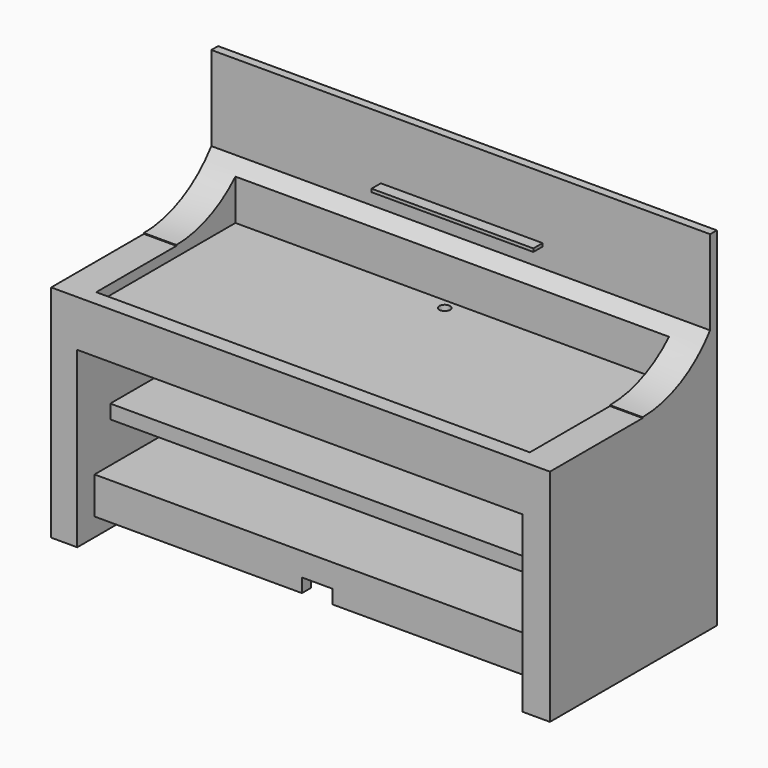
from build123d import *

# Parameters (mm, degrees)
F0_W          = 109.3183457851
F0_H          = 33.4434658289
F1_DEPTH      = 45.72
F2_W          = 95.0407683849
F2_H          = 38.138333708
F3_DEPTH      = 25.4
F4_W          = 109.3183457851
F4_H          = 23.2531316578
F5_DEPTH      = 25.4
F7_DEPTH      = 254
F9_W          = 5.9644132853
F9_H          = 45.72
F9_W_2        = 5.7119317353
F10_DEPTH     = 38.1
F11_W         = 29.130092822
F11_H         = 3.0559636652
F12_DEPTH     = 101.6
F14_DEPTH     = 127
F15_DEPTH     = 18.5456499457
F16_W         = 35.4631710798
F16_H         = 0.6852131337
F17_DEPTH     = 2.54
F18_W         = 38.6509299278
F18_H         = 8.1171598285
F19_DEPTH     = 99.9768525362
F20_T         = 2.54
F20_T3_DEPTH  = 114.3983457851
F20_T5_DEPTH  = 40.5431710798
F20_T7_DEPTH  = 5.7652131337
F20_T9_DEPTH  = 12.2003224361
F20_T11_DEPTH = 12.2372549641
F20_T13_DEPTH = 50.8
F20_T15_DEPTH = 13.1971598285
F20_T17_DEPTH = 43.7309299278
F20_T19_DEPTH = 34.210092822
F20_T21_DEPTH = 8.1359636652
F20_T23_DEPTH = 7.2268683422
F20_T25_DEPTH = 43.218333708
F20_T27_DEPTH = 14.0249238314
F20_T29_DEPTH = 100.1207683849
F21_W         = 6.7161731422
F21_H         = 3.0271708965
F22_DEPTH     = 25.4
F8_R          = 1.1732121366
F23_DEPTH     = 69.3976804614


# Not quite as in the source:
# - a shell that OpenCascade refuses in one call is made with other operations: the cavity is built on its own and cut out


with BuildPart() as f1:
    # F0 (on Front) → F1 (new body)
    with BuildSketch(Plane.XZ):
        with Locations((-0.1045018435, 16.7217329144)):
            Rectangle(F0_W, F0_H)
    extrude(amount=F1_DEPTH)

    # F2 (on face) → F3 (cut)
    with BuildSketch(Plane.XY.offset(33.4434658289)):
        with Locations((-0.1229681075, -23.2116412371)):
            Rectangle(F2_W, F2_H)
    extrude(amount=-F3_DEPTH, mode=Mode.SUBTRACT)

    # F4 (on face) → F5 (cut)
    with BuildSketch(Plane.XZ.offset(45.72)):
        with Locations((-0.1045018435, 21.8169)):
            Rectangle(F4_W, F4_H)
    extrude(amount=-F5_DEPTH, mode=Mode.SUBTRACT)

    # F6 (on face) → F7 (cut)
    with BuildSketch(Plane.YZ.offset(54.5546710491)):
        with BuildLine():
            Line((-20.32, 33.4434658289), (-20.32, 10.3678972162))
            ThreePointArc((-20.32, 10.3678972162), (-8.4847772871, 13.6341404962), (0, 22.5082261516))
            Line((0, 22.5082261516), (0, 33.4434658289))
            Line((0, 33.4434658289), (-20.32, 33.4434658289))
        make_face()
        with BuildLine():
            ThreePointArc((0, 22.5082261516), (2.0560745106, 27.8049237926), (2.7555686127, 33.4434658289))
            ThreePointArc((2.7555686127, 33.4434658289), (-36.6368910458, 49.7603568747), (-20.32, 10.3678972162))
            Line((-20.32, 10.3678972162), (-20.32, 33.4434658289))
            Line((-20.32, 33.4434658289), (0, 33.4434658289))
            Line((0, 33.4434658289), (0, 22.5082261516))
        make_face()
    extrude(amount=-F7_DEPTH, mode=Mode.SUBTRACT)

    # F9 (on face) → F10 (join)
    with BuildSketch(Plane(origin=(0, 0, 0), x_dir=(1, 0, 0), z_dir=(0, 0, -1))):
        with Locations((51.5724644065, 22.86)):
            Rectangle(F9_W, F9_H)
        with Locations((-51.9077088684, 22.86)):
            Rectangle(F9_W_2, F9_H)
    extrude(amount=F10_DEPTH)

    # F11 (on face) → F12 (join)
    with BuildSketch(Plane.YZ.offset(-49.0517430007)):
        with Locations((-22.1103844233, -15.5687723309)):
            Rectangle(F11_W, F11_H)
    extrude(amount=F12_DEPTH)

    # F13 (on face) → F14 (cut)
    with BuildSketch(Plane.YZ.offset(54.5546710491)):
        with BuildLine():
            ThreePointArc((0, 22.5082261516), (-0.8668457158, 21.0315096899), (-1.8408102843, 19.6231397021))
            Line((-1.8408102843, 19.6231397021), (0, 19.6231397021))
            Line((0, 19.6231397021), (0, 22.5082261516))
        make_face()
    extrude(amount=-F14_DEPTH, mode=Mode.SUBTRACT)

    # F15 (add): a face of the model
    f15_faces = [f1.faces().sort_by_distance(p)[0] for p in [
        (-0.1045018435, -0.9204051421, 19.6231397021),
    ]]
    extrude(f15_faces, amount=F15_DEPTH)

    # F16 (on face) → F17 (join)
    with BuildSketch(Plane.XZ.offset(1.8408102843)):
        with Locations((0.1093326136, 24.1770995781)):
            Rectangle(F16_W, F16_H)
    extrude(amount=F17_DEPTH)

    # F18 (on face) → F19 (join)
    with BuildSketch(Plane(origin=(48.5902577639, 0, 0), x_dir=(0, -1, 0), z_dir=(-1, 0, 0))):
        with Locations((21.6686017811, -30.0215007737)):
            Rectangle(F18_W, F18_H)
    extrude(amount=F19_DEPTH)

    # F20: shell of thickness 2.54, made by hand


with BuildPart() as f20_core1:
    # F20_t2: copy of F1
    add(f1.part)

    # the walls: a layer under each face that stays
    f20_faces = [f20_core1.faces().sort_by_distance(p)[0] for p in [
        (-54.763674736, -22.86, 0.0343948239),
        (-0.1045018435, 0, 0.0343948239),
        (-0.1045018435, -0.9204051421, 38.1687896479),
        (-0.1045018435, -1.8408102843, 28.895964675),
        (-46.9552214657, -2.7975084588, 18.4286678952),
        (-51.203513518, -20.32, 10.2791156936),
        (-46.9552214657, -43.9057142857, 10.1903341711),
        (-36.5439504385, -45.72, 2.1419451425),
        (-51.9077088684, -22.86, -38.1),
        (54.5546710491, -22.86, 0.0343948239),
        (-49.0517430007, -22.86, -19.05),
        (-0.2307426184, -22.86, 0),
        (48.5902577639, -22.86, -19.05),
        (51.5724644065, -22.86, -38.1),
        (0.1093326136, -3.1108102843, 24.5197061449),
        (-17.6222529262, -3.1108102843, 24.1770995781),
        (0.1093326136, -3.1108102843, 23.8344930112),
        (17.8409181535, -3.1108102843, 24.1770995781),
        (-47.6433522999, -10.4988633345, 9.5342864675),
        (-0.1229681075, -4.1424743831, 12.5159277446),
        (47.397416085, -35.9244191398, 9.5342864675),
        (50.9760435671, -20.32, 10.2791156936),
        (-0.1229681075, -42.2808080912, 9.1169),
        (-0.2307426184, -40.994066745, -30.0215007737),
        (-0.2307426184, -21.6686017811, -25.9629208595),
        (-0.2307426184, -2.3431368172, -30.0215007737),
        (-0.2307426184, -22.1103844233, -14.0407904983),
        (-0.2307426184, -7.5453380123, -15.5687723309),
        (-0.2307426184, -36.6754308343, -15.5687723309),
        (-0.2307426184, -22.1103844233, -17.0967541635),
        (0.1093326136, -4.3808102843, 24.1770995781),
        (-0.1229681075, -23.2116412371, 8.0434658289),
    ]]
    thicken(f20_faces, amount=-F20_T, mode=Mode.SUBTRACT)

    # F20_s4 → F20_t3 (cut)
    with BuildSketch(Plane.YZ.offset(-57.303674736)):
        Polygon((-1.8865509063, 19.6383521673), (0.6991897157, 19.6231397021), (0.6991897157, 18.7783837759), (0.1932519166, 18.1018931859), align=None)
    extrude(amount=F20_T3_DEPTH, mode=Mode.SUBTRACT)

    # F20_s6 → F20_t5 (cut)
    with BuildSketch(Plane.YZ.offset(-20.1622529262)):
        Polygon((-1.8662102843, 24.5451061449), (0.6991897157, 24.5197061449), (0.6991897157, 21.9797061449), (-1.8408102843, 21.9797061449), align=None)
        Polygon((-1.8662102843, 23.8090930112), (0.6991897157, 23.8344930112), (0.6991897157, 26.3744930112), (-1.8408102843, 26.3744930112), align=None)
    extrude(amount=F20_T5_DEPTH, mode=Mode.SUBTRACT)

    # F20_s8 → F20_t7 (cut)
    with BuildSketch(Plane.XY.offset(21.2944930112)):
        Polygon((-17.6476529262, -1.8662102843), (-17.6222529262, 0.6991897157), (-15.0822529262, 0.6991897157), (-15.0822529262, -1.8408102843), align=None)
        Polygon((17.8663181535, -1.8662102843), (17.8409181535, 0.6991897157), (15.3009181535, 0.6991897157), (15.3009181535, -1.8408102843), align=None)
    extrude(amount=F20_T7_DEPTH, mode=Mode.SUBTRACT)

    # F20_s10 → F20_t9 (cut)
    with BuildSketch(Plane.YZ.offset(-57.303674736)):
        Polygon((-20.3454, 10.2157341711), (-17.78, 10.1903341711), (-17.78, 7.6503341711), (-20.32, 7.6503341711), align=None)
    extrude(amount=F20_T9_DEPTH, mode=Mode.SUBTRACT)

    # F20_s12 → F20_t11 (cut)
    with BuildSketch(Plane.YZ.offset(44.857416085)):
        Polygon((-20.3454, 10.2157341711), (-20.32, 7.6503341711), (-17.78, 7.6503341711), (-17.78, 10.1903341711), align=None)
    extrude(amount=F20_T11_DEPTH, mode=Mode.SUBTRACT)

    # F20_s14 → F20_t13 (cut)
    with BuildSketch(Plane.XZ.offset(-2.54)):
        Polygon((-49.0263430007, -0.0254), (-51.5917430007, 0), (-51.5917430007, 2.54), (-49.0517430007, 2.54), align=None)
        Polygon((48.5648577639, -0.0254), (48.5902577639, 2.54), (51.1302577639, 2.54), (51.1302577639, 0), align=None)
    extrude(amount=F20_T13_DEPTH, mode=Mode.SUBTRACT)

    # F20_s16 → F20_t15 (cut)
    with BuildSketch(Plane.XY.offset(-36.620080688)):
        Polygon((-49.0263430007, -41.019466745), (-51.5917430007, -40.994066745), (-51.5917430007, -38.454066745), (-49.0517430007, -38.454066745), align=None)
        Polygon((-49.0263430007, -2.3177368172), (-51.5917430007, -2.3431368172), (-51.5917430007, -4.8831368172), (-49.0517430007, -4.8831368172), align=None)
        Polygon((48.5648577639, -2.3177368172), (51.1302577639, -2.3431368172), (51.1302577639, -4.8831368172), (48.5902577639, -4.8831368172), align=None)
        Polygon((48.5648577639, -41.019466745), (51.1302577639, -40.994066745), (51.1302577639, -38.454066745), (48.5902577639, -38.454066745), align=None)
    extrude(amount=F20_T15_DEPTH, mode=Mode.SUBTRACT)

    # F20_s18 → F20_t17 (cut)
    with BuildSketch(Plane.XZ.offset(-0.1968631828)):
        Polygon((-49.0263430007, -25.9375208595), (-51.5917430007, -25.9629208595), (-51.5917430007, -28.5029208595), (-49.0517430007, -28.5029208595), align=None)
        Polygon((48.5648577639, -25.9375208595), (51.1302577639, -25.9629208595), (51.1302577639, -28.5029208595), (48.5902577639, -28.5029208595), align=None)
    extrude(amount=F20_T17_DEPTH, mode=Mode.SUBTRACT)

    # F20_s20 → F20_t19 (cut)
    with BuildSketch(Plane.XZ.offset(5.0053380123)):
        Polygon((-49.0263430007, -14.0153904983), (-51.5917430007, -14.0407904983), (-51.5917430007, -16.5807904983), (-49.0517430007, -16.5807904983), align=None)
        Polygon((-49.0263430007, -17.1221541635), (-51.5917430007, -17.0967541635), (-51.5917430007, -14.5567541635), (-49.0517430007, -14.5567541635), align=None)
        Polygon((48.5648577639, -17.1221541635), (51.1302577639, -17.0967541635), (51.1302577639, -14.5567541635), (48.5902577639, -14.5567541635), align=None)
        Polygon((48.5648577639, -14.0153904983), (51.1302577639, -14.0407904983), (51.1302577639, -16.5807904983), (48.5902577639, -16.5807904983), align=None)
    extrude(amount=F20_T19_DEPTH, mode=Mode.SUBTRACT)

    # F20_s22 → F20_t21 (cut)
    with BuildSketch(Plane.XY.offset(-19.6367541635)):
        Polygon((-49.0263430007, -7.5199380123), (-51.5917430007, -7.5453380123), (-51.5917430007, -10.0853380123), (-49.0517430007, -10.0853380123), align=None)
        Polygon((-49.0263430007, -36.7008308343), (-51.5917430007, -36.6754308343), (-51.5917430007, -34.1354308343), (-49.0517430007, -34.1354308343), align=None)
        Polygon((48.5648577639, -7.5199380123), (51.1302577639, -7.5453380123), (51.1302577639, -10.0853380123), (48.5902577639, -10.0853380123), align=None)
        Polygon((48.5648577639, -36.7008308343), (51.1302577639, -36.6754308343), (51.1302577639, -34.1354308343), (48.5902577639, -34.1354308343), align=None)
    extrude(amount=F20_T21_DEPTH, mode=Mode.SUBTRACT)

    # F20_s24 → F20_t23 (cut)
    with BuildSketch(Plane.XY.offset(5.5034658289)):
        Polygon((-47.6179522999, -42.2554080912), (-50.1833522999, -42.2808080912), (-50.1833522999, -44.8208080912), (-47.6433522999, -44.8208080912), align=None)
        Polygon((47.372016085, -42.2554080912), (49.937416085, -42.2808080912), (49.937416085, -44.8208080912), (47.397416085, -44.8208080912), align=None)
    extrude(amount=F20_T23_DEPTH, mode=Mode.SUBTRACT)

    # F20_s26 → F20_t25 (cut)
    with BuildSketch(Plane.XZ.offset(1.6024743831)):
        Polygon((-47.6179522999, 8.0688658289), (-50.1833522999, 8.0434658289), (-50.1833522999, 5.5034658289), (-47.6433522999, 5.5034658289), align=None)
        Polygon((47.372016085, 8.0688658289), (49.937416085, 8.0434658289), (49.937416085, 5.5034658289), (47.397416085, 5.5034658289), align=None)
    extrude(amount=F20_T25_DEPTH, mode=Mode.SUBTRACT)

    # F20_s28 → F20_t27 (cut)
    with BuildSketch(Plane.XY.offset(5.5034658289)):
        Polygon((-47.6179522999, -4.1678743831), (-50.1833522999, -4.1424743831), (-50.1833522999, -1.6024743831), (-47.6433522999, -1.6024743831), align=None)
        Polygon((47.372016085, -4.1678743831), (47.397416085, -1.6024743831), (49.937416085, -1.6024743831), (49.937416085, -4.1424743831), align=None)
    extrude(amount=F20_T27_DEPTH, mode=Mode.SUBTRACT)

    # F20_s30 → F20_t29 (cut)
    with BuildSketch(Plane.YZ.offset(-50.1833522999)):
        Polygon((-4.1678743831, 8.0688658289), (-1.6024743831, 8.0434658289), (-1.6024743831, 5.5034658289), (-4.1424743831, 5.5034658289), align=None)
        Polygon((-42.2554080912, 8.0688658289), (-44.8208080912, 8.0434658289), (-44.8208080912, 5.5034658289), (-42.2808080912, 5.5034658289), align=None)
    extrude(amount=F20_T29_DEPTH, mode=Mode.SUBTRACT)


with BuildPart() as f1_1:
    add(f1.part)

    # what is left inside the walls is the cavity
    f20_cavity = [f20_core1.part.solids().sort_by_distance(p)[0] for p in [
        (-0.230743, -29.633333, 2.5654),
    ]]
    add(f20_cavity, mode=Mode.SUBTRACT)

    # F21 (on face) → F22 (cut)
    with BuildSketch(Plane.XZ.offset(40.994066745)):
        with Locations((-0.2307426184, -32.5664952397)):
            Rectangle(F21_W, F21_H)
    extrude(amount=-F22_DEPTH, mode=Mode.SUBTRACT)

    # F8 (on face) → F23 (cut)
    with BuildSketch(Plane.XY.offset(8.0434658289)):
        with Locations((0, -6.3559673727)):
            Circle(F8_R)
    extrude(amount=-F23_DEPTH, mode=Mode.SUBTRACT)


solid = f1_1.part
